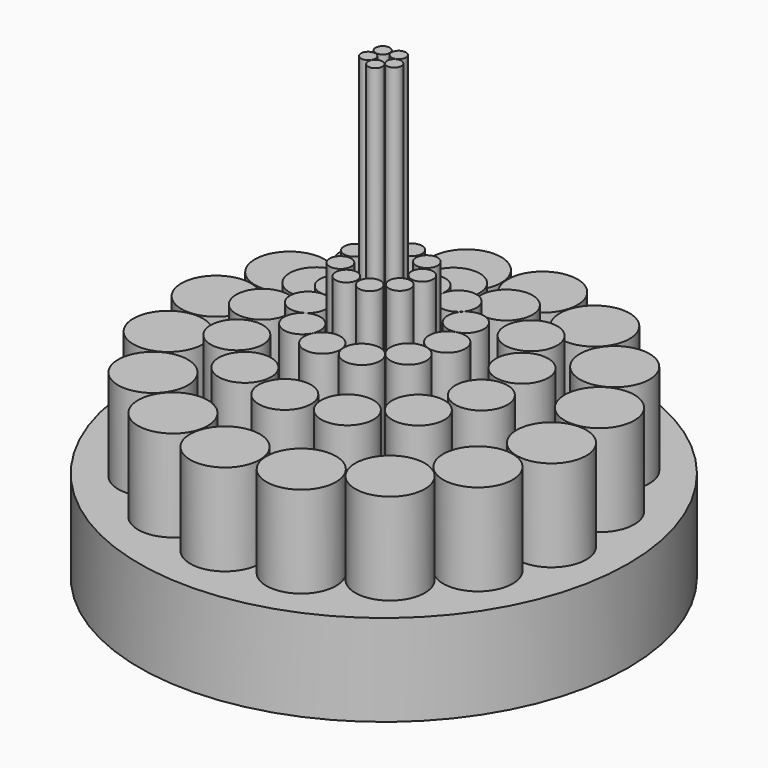
from build123d import *

# Parameters (mm, degrees)
F0_R             = 67.8801752346
F1_DEPTH         = 12.7
F2_R             = 9.6644171041
F3_DEPTH         = 25.4
F3_COPIES_COUNT  = 16
F4_R             = 7.2675454898
F5_DEPTH         = 31.75
F5_COPIES_COUNT  = 13
F6_R             = 5.0242913047
F7_DEPTH         = 38.1
F7_COPIES_COUNT  = 11
F8_R             = 3.0016652879
F9_DEPTH         = 50.8
F9_COPIES_COUNT  = 9
F10_R            = 1.9805186859
F11_DEPTH        = 101.6
F11_COPIES_COUNT = 5


# Not quite as in the source:
# - a pattern or mirror of a feature is missing from the dataset's text; its kind, count and spacing are read off the source's solid


with BuildPart() as f1:
    # F0 (on Top) → F1 (new body, symmetric)
    with BuildSketch(Plane.XY):
        Circle(F0_R)
    extrude(amount=F1_DEPTH, both=True)

    # F2 (on face) → F3 (join)
    with BuildSketch(Plane.XY.offset(12.7)):
        with Locations((-32.3193110526, 38.2313802838)):
            Circle(F2_R)
    f3 = extrude(amount=F3_DEPTH)

    # F3_copies: F3 ×16 about axis
    f3_copies_axis = Axis((0, 0, 0), (0, 0, 1))
    for i in range(1, F3_COPIES_COUNT):
        add(f3.rotate(f3_copies_axis, i * 360 / F3_COPIES_COUNT))

    # F4 (on face) → F5 (join)
    with BuildSketch(Plane.XY.offset(12.7)):
        with Locations((-19.9039652944, 25.22482723)):
            Circle(F4_R)
    f5 = extrude(amount=F5_DEPTH)

    # F5_copies: F5 ×13 about axis
    f5_copies_axis = Axis((0, 0, 0), (0, 0, 1))
    for i in range(1, F5_COPIES_COUNT):
        add(f5.rotate(f5_copies_axis, i * 360 / F5_COPIES_COUNT))

    # F6 (on face) → F7 (join)
    with BuildSketch(Plane.XY.offset(12.7)):
        with Locations((-11.4300008863, 13.7948282063)):
            Circle(F6_R)
    f7 = extrude(amount=F7_DEPTH)

    # F7_copies: F7 ×11 about axis
    f7_copies_axis = Axis((0, 0, 0), (0, 0, 1))
    for i in range(1, F7_COPIES_COUNT):
        add(f7.rotate(f7_copies_axis, i * 360 / F7_COPIES_COUNT))

    # F8 (on face) → F9 (join)
    with BuildSketch(Plane.XY.offset(12.7)):
        with Locations((-6.1091380194, 7.2915516794)):
            Circle(F8_R)
    f9 = extrude(amount=F9_DEPTH)

    # F9_copies: F9 ×9 about axis
    f9_copies_axis = Axis((0, 0, 0), (0, 0, 1))
    for i in range(1, F9_COPIES_COUNT):
        add(f9.rotate(f9_copies_axis, i * 360 / F9_COPIES_COUNT))

    # F10 (on face) → F11 (join)
    with BuildSketch(Plane.XY.offset(12.7)):
        with Locations((-2.36482732, 2.5618965738)):
            Circle(F10_R)
    f11 = extrude(amount=F11_DEPTH)

    # F11_copies: F11 ×5 about axis
    f11_copies_axis = Axis((0, 0, 0), (0, 0, 1))
    for i in range(1, F11_COPIES_COUNT):
        add(f11.rotate(f11_copies_axis, i * 360 / F11_COPIES_COUNT))


solid = f1.part
